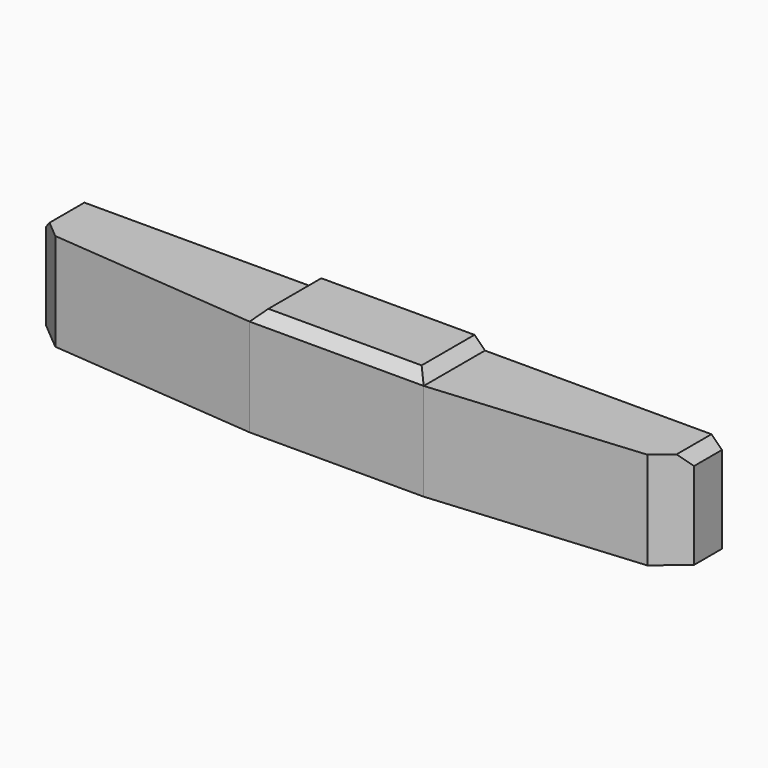
from build123d import *

# Parameters (mm, degrees)
F1_DEPTH = 355.6
F2_W     = 635
F2_H     = 279.345146747
F3_DEPTH = 38.1
F4_SIZE  = 38.09999
F5_SIZE  = 38.1


# Not quite as in the source:
# - a fillet or chamfer is up to 0.001 mm smaller than in the source, because OpenCascade refuses the exact size


with BuildPart() as f1:
    # F0 (on Top) → F1 (new body)
    with BuildSketch(Plane.XY):
        Polygon((2363.263666194, 0), (0, 0), (0, -127), (102.108, -212.6787851403), (864.108, -279.345146747), (1499.108, -279.345146747), (2261.108, -212.7113899342), (2363.263666194, -127), align=None)
    extrude(amount=F1_DEPTH)

    # F2 (on face) → F3 (join)
    with BuildSketch(Plane.XY.offset(355.6)):
        with Locations((1181.608, -139.6725733735)):
            Rectangle(F2_W, F2_H)
    extrude(amount=F3_DEPTH)

    # F4 (size 38.1 in the source; OpenCascade refuses exactly that, so slightly less here)
    f4_edges = [f1.edges().sort_by_distance(p)[0] for p in [
        (864.108, -139.672573, 393.7),
        (1499.108, -139.672573, 393.7),
    ]]
    chamfer(f4_edges, length=F4_SIZE)

    # F5
    f5_edges = [f1.edges().sort_by_distance(p)[0] for p in [
        (0, -63.5, 355.6),
        (1181.608, -279.345147, 393.7),
        (2363.263666, -63.5, 355.6),
    ]]
    chamfer(f5_edges, length=F5_SIZE)


solid = f1.part
